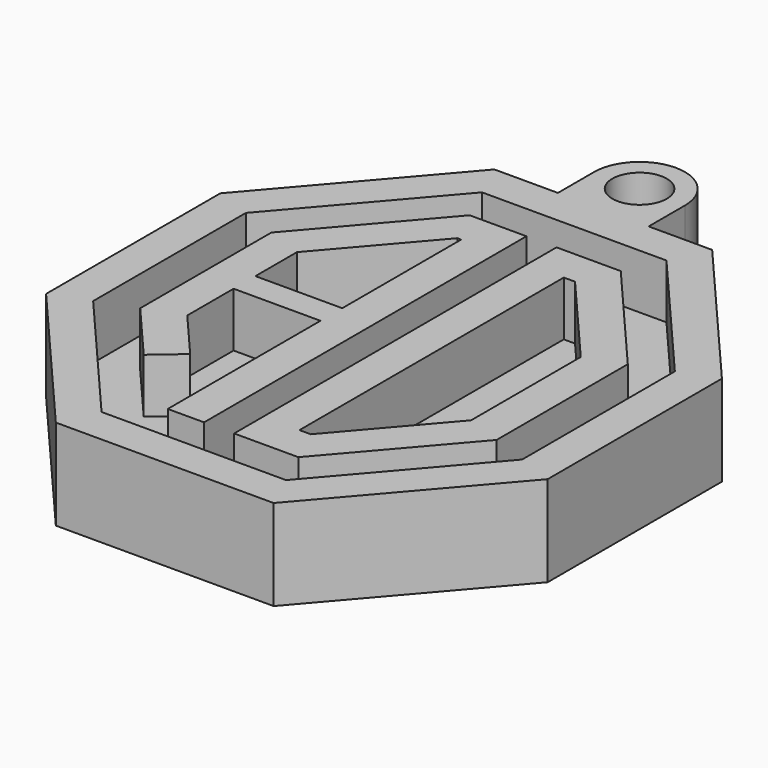
from build123d import *

# Parameters (mm, degrees)
F1_DEPTH  = 5
F3_DEPTH  = 3
F5_DEPTH  = 3
F7_DEPTH  = 5
F8_R      = 2.49999
F9_R      = 1.5
F10_DEPTH = 5


# Not quite as in the source:
# - a fillet or chamfer is up to 0.001 mm smaller than in the source, because OpenCascade refuses the exact size


with BuildPart() as f1:
    # F0 (on Top) → F1 (new body)
    with BuildSketch(Plane.XY):
        Polygon((0, 6), (0, 0), (7.8194713464, -9.1025198634), (13.8194713464, -9.1025198634), (19.8194713464, -9.1025198634), (27.6389426928, 0), (27.6389426928, 6), (27.6389426928, 12), (19.8194713464, 21.1025198634), (13.8194713464, 21.1025198634), (7.8194713464, 21.1025198634), (0, 12), align=None)
    extrude(amount=F1_DEPTH)

    # F2 (on face) → F3 (cut)
    with BuildSketch(Plane.XY.offset(5)):
        Polygon((2, 11.2589063868), (2, 0.7410936132), (8.7380145007, -7.1025198634), (18.9009281921, -7.1025198634), (25.6389426928, 0.7410936132), (25.6389426928, 11.2589063868), (18.9009281921, 19.1025198634), (8.7380145007, 19.1025198634), align=None)
    extrude(amount=-F3_DEPTH, mode=Mode.SUBTRACT)

    # F4 (on face) → F5 (join)
    with BuildSketch(Plane.XY.offset(2)):
        Polygon((17.9823850378, -5.1025198634), (23.6389426928, 1.4821872264), (23.6389426928, 10.5178127736), (17.9823850378, 17.1025198634), (14.4432382658, 17.1025198634), (14.4432382658, -5.1025198634), align=None)
        Polygon((16.4432382658, -3.1025198634), (16.4432382658, 15.1025198634), (17.0638418835, 15.1025198634), (21.6389426928, 9.7767191605), (21.6389426928, 2.2232808395), (17.0638418835, -3.1025198634), align=None, mode=Mode.SUBTRACT)
        Polygon((10.7860844582, -3.1025198634), (10.7860844582, -5.1025198634), (12.7860844582, -5.1025198634), (12.7860844582, 17.1025198634), (9.6565576549, 17.1025198634), (4, 10.5178127736), (4, 1.4821872264), (6.8282788275, -1.8101663185), (8.3453654714, -0.5069210941), (6, 2.2232808395), (6, 5.4149306379), (10.7860844582, 5.4149306379), align=None)
        Polygon((6, 9.7767191605), (10.5751008092, 15.1025198634), (10.7860844582, 15.1025198634), (10.7860844582, 6.9169756025), (6, 6.9169756025), align=None, mode=Mode.SUBTRACT)
    extrude(amount=F5_DEPTH)

    # F6 (on face) → F7 (join)
    with BuildSketch(Plane(origin=(0, 21.1025198634, 0), x_dir=(-1, 0, 0), z_dir=(0, 1, 0))):
        Polygon((-11.3194713464, 5), (-13.8194713464, 5), (-16.3194713464, 5), (-16.3194713464, 0), (-11.3194713464, 0), align=None)
    extrude(amount=F7_DEPTH)

    # F8 (radius 2.5 in the source; OpenCascade refuses exactly that, so slightly less here)
    f8_edges = [f1.edges().sort_by_distance(p)[0] for p in [
        (11.319471, 26.10252, 2.5),
        (16.319471, 26.10252, 2.5),
    ]]
    fillet(f8_edges, radius=F8_R)

    # F9 (on face) → F10 (cut)
    with BuildSketch(Plane.XY.offset(5)):
        with Locations((13.8194713464, 23.6025198634)):
            Circle(F9_R)
    extrude(amount=-F10_DEPTH, mode=Mode.SUBTRACT)


solid = f1.part
